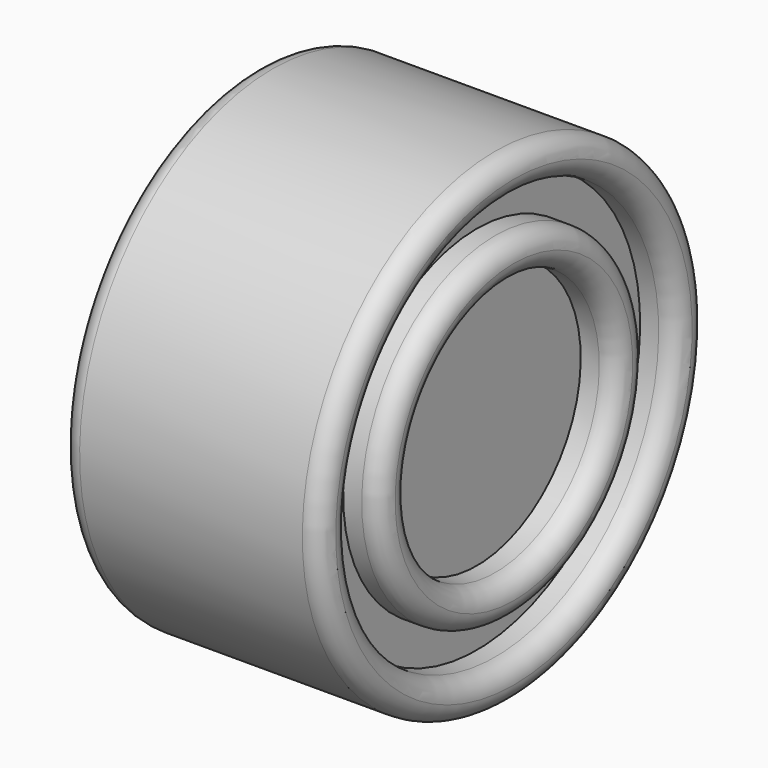
from build123d import *

# Parameters (mm, degrees)
F0_W     = 2
F0_H     = 2
F0_W_2   = 12
F2_R     = 0.99999
F3_R     = 1.4
F4_DEPTH = 10


# Not quite as in the source:
# - a fillet or chamfer is up to 0.001 mm smaller than in the source, because OpenCascade refuses the exact size


with BuildPart() as f1:
    # F0 (on Front) → F1 (revolve)
    with BuildSketch(Plane.XZ):
        Polygon((-12, 0), (0, 0), (0, 7), (0, 9), (0, 11), (-12, 11), align=None)
        with Locations((1, 8)):
            Rectangle(F0_W, F0_H)
        with Locations((-6, 12)):
            Rectangle(F0_W_2, F0_H)
        with Locations((1, 12)):
            Rectangle(F0_W, F0_H)
    revolve(axis=Axis((-6, 0, 0), (-1, 0, 0)))

    # F2 (radius 1 in the source; OpenCascade refuses exactly that, so slightly less here)
    f2_edges = [f1.edges().sort_by_distance(p)[0] for p in [
        (2, 0, -13),
        (2, 0, -9),
        (2, 0, -7),
        (2, 0, -11),
        (-12, 0, -13),
    ]]
    fillet(f2_edges, radius=F2_R)

    # F3 (on face) → F4 (cut)
    with BuildSketch(Plane(origin=(-12, 0, 0), x_dir=(0, -1, 0), z_dir=(-1, 0, 0))):
        Circle(F3_R)
    extrude(amount=-F4_DEPTH, mode=Mode.SUBTRACT)


solid = f1.part
